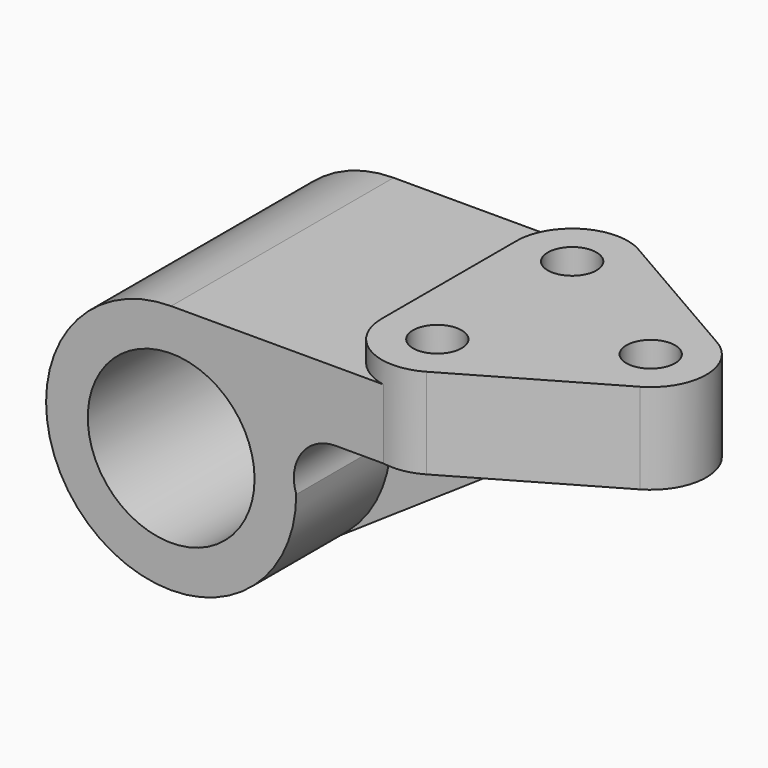
from build123d import *

# Parameters (mm, degrees)
F0_R     = 19.05
F1_DEPTH = 31.75
F4_R     = 5.5626
F5_DEPTH = 20.6502
F6_DEPTH = 20.6512
F8_DEPTH = 4.7625


with BuildPart() as f1:
    # F0 (on Front) → F1 (new body, symmetric)
    with BuildSketch(Plane.XZ):
        with BuildLine():
            ThreePointArc((28.575, 0), (29.7781261877, 8.674261314), (37.5552561211, 12.7))
            Line((37.5552561211, 12.7), (50.8, 12.7))
            Line((50.8, 12.7), (50.8, 28.575))
            Line((50.8, 28.575), (0, 28.575))
            ThreePointArc((0, 28.575), (-20.2055762724, -20.2055762724), (28.575, 0))
        make_face()
        Circle(F0_R, mode=Mode.SUBTRACT)
    extrude(amount=F1_DEPTH, both=True)

    # F4 (on face) → F5 (join)
    with BuildSketch(Plane(origin=(0, 0, 12.7), x_dir=(1, 0, 0), z_dir=(0, 0, -1))):
        with BuildLine():
            ThreePointArc((90.5002, -10.9985226281), (96.8502, 0), (90.5002, 10.9985226281))
            Line((90.5002, 10.9985226281), (57.15, 30.2532695756))
            ThreePointArc((57.15, 30.2532695756), (44.45, 30.2532695756), (38.1, 19.2547469475))
            Line((38.1, 19.2547469475), (38.1, -19.2547469475))
            ThreePointArc((38.1, -19.2547469475), (44.45, -30.2532695756), (57.15, -30.2532695756))
            Line((57.15, -30.2532695756), (90.5002, -10.9985226281))
        make_face()
        with Locations((50.8, -19.2547469475)):
            Circle(F4_R, mode=Mode.SUBTRACT)
        with Locations((50.8, 19.2547469475)):
            Circle(F4_R, mode=Mode.SUBTRACT)
        with Locations((84.1502, 0)):
            Circle(F4_R, mode=Mode.SUBTRACT)
    extrude(amount=-F5_DEPTH)

    # F4 (on face) → F6 (cut, through all)
    with BuildSketch(Plane(origin=(0, 0, 12.7), x_dir=(1, 0, 0), z_dir=(0, 0, -1))):
        with BuildLine():
            Line((50.8, 13.6921469475), (50.8, 24.8173469475))
            ThreePointArc((50.8, 24.8173469475), (45.2374, 19.2547469475), (50.8, 13.6921469475))
        make_face()
        with BuildLine():
            ThreePointArc((50.8, -13.6921469475), (45.2374, -19.2547469475), (50.8, -24.8173469475))
            Line((50.8, -24.8173469475), (50.8, -13.6921469475))
        make_face()
    extrude(amount=-F6_DEPTH, mode=Mode.SUBTRACT)

    # F7 (on Front) → F8 (join, symmetric)
    with BuildSketch(Plane.XZ):
        with BuildLine():
            Line((48.5287335791, 12.7), (37.5552561211, 12.7))
            ThreePointArc((37.5552561211, 12.7), (29.7781261877, 8.674261314), (28.575, 0))
            ThreePointArc((28.575, 0), (25.2347822744, -13.4065800472), (15.9950252975, -23.6788891364))
            Line((15.9950252975, -23.6788891364), (69.85, 12.7))
            Line((69.85, 12.7), (57.15, 12.7))
            Line((57.15, 12.7), (48.5287335791, 12.7))
        make_face()
    extrude(amount=F8_DEPTH, both=True)


solid = f1.part
